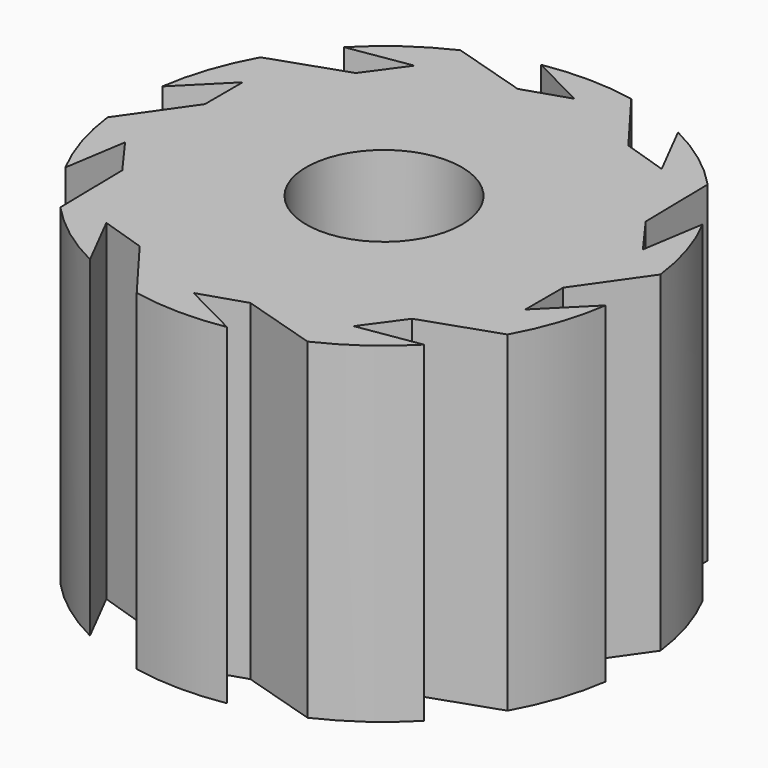
from build123d import *

# Parameters (mm, degrees)
F2_R            = 9.525
F2_R_2          = 2.921
F3_DEPTH        = 12.446
F5_DEPTH        = 12.446
F5_COPIES_COUNT = 10


# Not quite as in the source:
# - a pattern or mirror of a feature is missing from the dataset's text; its kind, count and spacing are read off the source's solid


with BuildPart() as f3:
    # F2 (on Top) → F3 (new body)
    with BuildSketch(Plane.XY):
        Circle(F2_R)
        Circle(F2_R_2, mode=Mode.SUBTRACT)
    extrude(amount=F3_DEPTH)

    # F4 (on face) → F5 (cut, through all)
    with BuildSketch(Plane.XY.offset(12.446)):
        Polygon((9.525, -1.27), (9.525, 1.27), (7.747, -1.269247156), (7.747, -3.048), align=None)
    f5 = extrude(amount=-F5_DEPTH, mode=Mode.SUBTRACT)

    # F5_copies: F5 ×10 about axis
    f5_copies_axis = Axis((0, 0, 0), (0, 0, 1))
    for i in range(1, F5_COPIES_COUNT):
        add(f5.rotate(f5_copies_axis, i * 360 / F5_COPIES_COUNT), mode=Mode.SUBTRACT)


solid = f3.part
